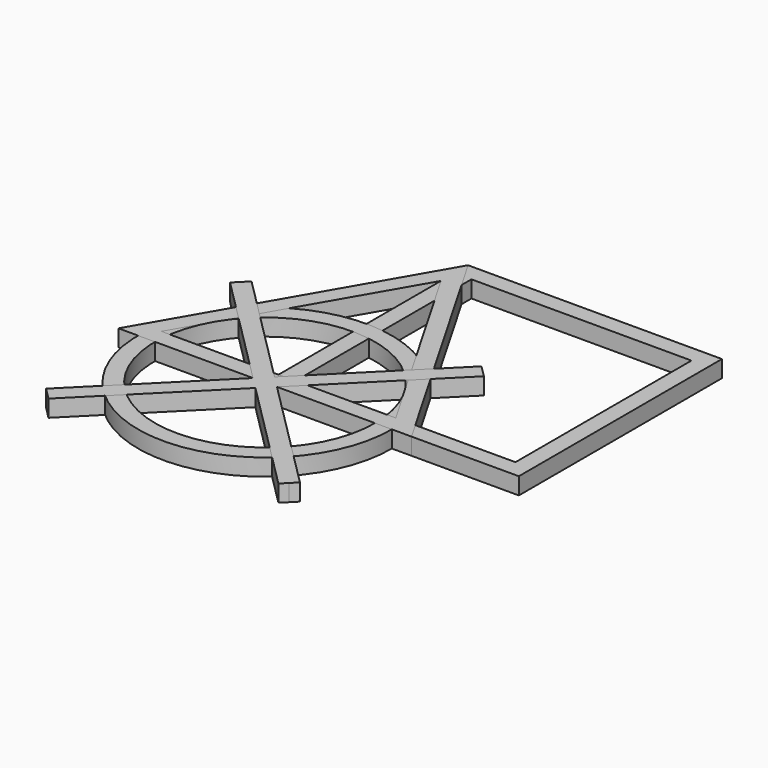
from build123d import *

# Parameters (mm, degrees)
F0_W     = 150
F0_H     = 150
F0_W_2   = 130
F0_H_2   = 130
F1_DEPTH = 10
F3_R     = 75
F3_R_2   = 65
F4_DEPTH = 10
F5_DEPTH = 10
F7_DEPTH = 10
F9_COUNT = 4


with BuildPart() as f1:
    # F0 (on Top) → F1 (new body)
    with BuildSketch(Plane.XY):
        with Locations((75, 75)):
            Rectangle(F0_W, F0_H)
        with Locations((75, 75)):
            Rectangle(F0_W_2, F0_H_2, mode=Mode.SUBTRACT)
    extrude(amount=F1_DEPTH)


with BuildPart() as f4:
    # F3 (on Top) → F4 (new body)
    with BuildSketch(Plane.XY):
        Circle(F3_R)
        Circle(F3_R_2, mode=Mode.SUBTRACT)
    extrude(amount=F4_DEPTH)


with BuildPart() as f5:
    # F2 (on Top) → F5 (new body)
    with BuildSketch(Plane.XY):
        Polygon((86.6025403784, 0), (0, 150), (-86.6025403784, 0), align=None)
        Polygon((-69.2820323028, 10), (0, 130), (69.2820323028, 10), align=None, mode=Mode.SUBTRACT)
    extrude(amount=F5_DEPTH)


with BuildPart() as f7:
    # F6 (on Top) → F7 (new body)
    with BuildSketch(Plane.XY):
        Polygon((75, 67.9289321881), (71.4644660941, 71.4644660941), (67.9289321881, 75), (-3.5355339059, 3.5355339059), (0, 0), (3.5355339059, -3.5355339059), align=None)
    extrude(amount=F7_DEPTH)

    # F9: F7 ×4 about axis
    f9_axis = Axis((0, 0, 5), (0, 0, 1))


with BuildPart() as f7_1:
    add(f7.part)
    for i in range(1, F9_COUNT):
        add(f7.part.rotate(f9_axis, i * 360 / F9_COUNT))


solid = Compound([f1.part, f4.part, f5.part, f7_1.part])
